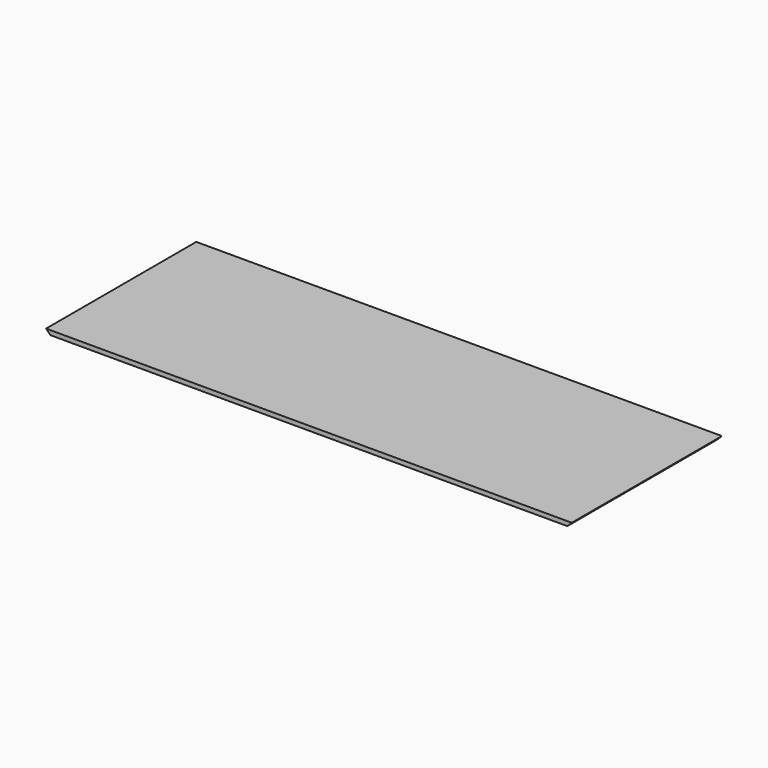
from build123d import *

# Parameters (mm, degrees)
F0_W     = 2133.6
F0_H     = 762
F1_DEPTH = 17.99844
F2_SIZE  = 17.99843


# Not quite as in the source:
# - a fillet or chamfer is up to 0.001 mm smaller than in the source, because OpenCascade refuses the exact size


with BuildPart() as f1:
    # F0 (on Top) → F1 (new body)
    with BuildSketch(Plane.XY):
        with Locations((1066.8, 381)):
            Rectangle(F0_W, F0_H)
    extrude(amount=-F1_DEPTH)

    # F2 (size 17.99844 in the source; OpenCascade refuses exactly that, so slightly less here)
    f2_edges = [f1.edges().sort_by_distance(p)[0] for p in [
        (2133.6, 381, -17.99844),
        (0, 381, -17.99844),
    ]]
    chamfer(f2_edges, length=F2_SIZE)


solid = f1.part
